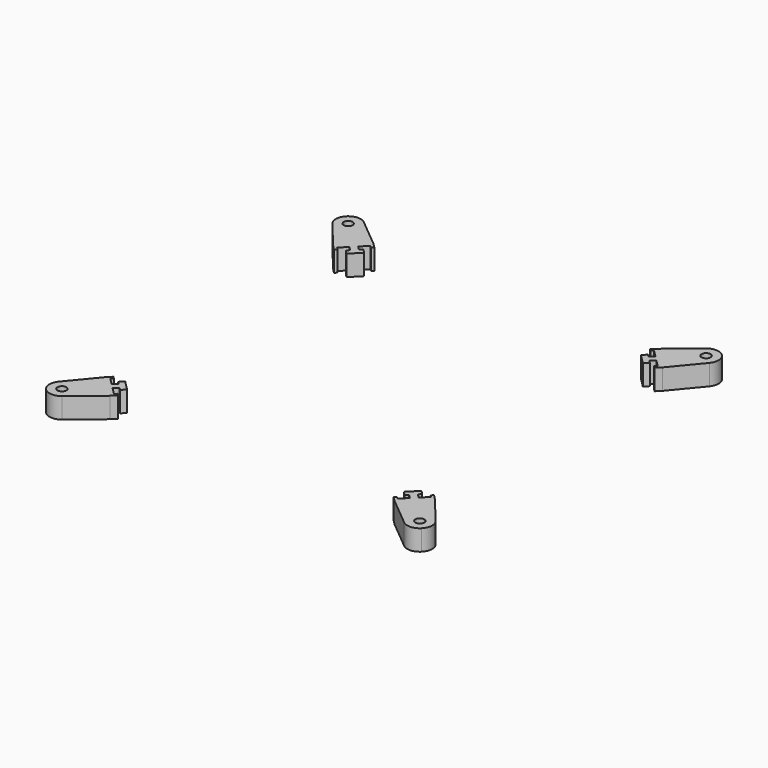
from build123d import *

# Parameters (mm, degrees)
F3_R            = 3.25
F4_DEPTH        = 15
F4_COPIES_COUNT = 4


# Not quite as in the source:
# - a pattern or mirror of a feature is missing from the dataset's text; its kind, count and spacing are read off the source's solid


with BuildPart() as f4:
    # F3 (on offset) → F4 (new body)
    with BuildSketch(Plane.XY.offset(5)):
        with BuildLine():
            Line((107.4802307404, -100.4091629285), (100.4091629285, -107.4802307404))
            Line((100.4091629285, -107.4802307404), (103.2375900532, -110.3086578651))
            Line((103.2375900532, -110.3086578651), (105.0053570062, -108.5408909121))
            Line((105.0053570062, -108.5408909121), (107.8337841309, -111.3693180369))
            Line((107.8337841309, -111.3693180369), (102.8840366626, -116.3190655052))
            Line((102.8840366626, -116.3190655052), (101.4698231003, -114.9048519428))
            Line((101.4698231003, -114.9048519428), (100.0556095379, -116.3190655052))
            Line((100.0556095379, -116.3190655052), (103.2375900532, -119.5010460205))
            Line((103.2375900532, -119.5010460205), (124.0861280516, -136.757884182))
            ThreePointArc((124.0861280516, -136.757884182), (130.2475566054, -138.8148707154), (136.1887660565, -136.1887660565))
            ThreePointArc((136.1887660565, -136.1887660565), (138.8148707154, -130.2475566054), (136.757884182, -124.0861280516))
            Line((136.757884182, -124.0861280516), (119.5010460205, -103.2375900532))
            Line((119.5010460205, -103.2375900532), (116.3190655052, -100.0556095379))
            Line((116.3190655052, -100.0556095379), (114.9048519428, -101.4698231003))
            Line((114.9048519428, -101.4698231003), (116.3190655052, -102.8840366626))
            Line((116.3190655052, -102.8840366626), (111.3693180369, -107.8337841309))
            Line((111.3693180369, -107.8337841309), (108.5408909121, -105.0053570062))
            Line((108.5408909121, -105.0053570062), (110.3086578651, -103.2375900532))
            Line((110.3086578651, -103.2375900532), (107.4802307404, -100.4091629285))
        make_face()
        with Locations((129.8248050259, -129.8248050259)):
            Circle(F3_R, mode=Mode.SUBTRACT)
    extrude(amount=F4_DEPTH)


with BuildPart() as f4_copies_1:
    # F4_copies: instance of F4
    add(f4.part.rotate(Axis((0, 0, 0), (0, 0, 1)), 1 * 360 / F4_COPIES_COUNT))


with BuildPart() as f4_copies_2:
    # F4_copies: instance of F4
    add(f4.part.rotate(Axis((0, 0, 0), (0, 0, 1)), 2 * 360 / F4_COPIES_COUNT))


with BuildPart() as f4_copies_3:
    # F4_copies: instance of F4
    add(f4.part.rotate(Axis((0, 0, 0), (0, 0, 1)), 3 * 360 / F4_COPIES_COUNT))


solid = Compound([f4.part, f4_copies_1.part, f4_copies_2.part, f4_copies_3.part])
